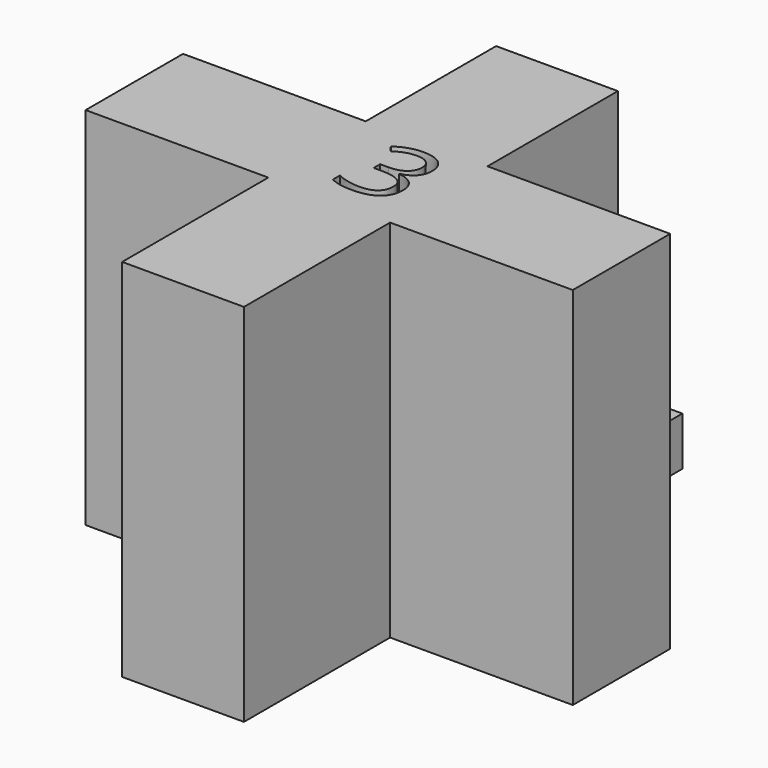
from build123d import *

# Parameters (mm, degrees)
F0_W         = 12.7
F0_H         = 57.15
F1_DEPTH     = 5.08
F2_W         = 50.8
F2_H         = 12.7
F3_DEPTH     = 38.1
F4_W         = 12.7
F4_H         = 48.7413735385
F5_DEPTH     = 33.02
F6_TEXT_SIZE = 12.0747026004
F7_DEPTH     = 2.54


# Not quite as in the source:
# - Text() gives the source's letters only with a copy of the font that has no kerning and outlines rounded to 1/6400 em; it was checked with that copy


with BuildPart() as f1:
    # F0 (on Top) → F1 (new body)
    with BuildSketch(Plane.XY):
        with Locations((-37.0165128261, 2.9978602284)):
            Rectangle(F0_W, F0_H)
    extrude(amount=F1_DEPTH)

    # F2 (on Top) → F3 (join)
    with BuildSketch(Plane.XY):
        with Locations((-37.0165128261, -0.1771397716)):
            Rectangle(F2_W, F2_H)
    extrude(amount=F3_DEPTH)

    # F4 (on face) → F5 (join)
    with BuildSketch(Plane.XY.offset(5.08)):
        with Locations((-37.0165128261, -1.2064530024)):
            Rectangle(F4_W, F4_H)
    extrude(amount=F5_DEPTH)

    # F6 (on face) → F7 (cut)
    with BuildSketch(Plane.XY.offset(38.1)):
        with Locations((-39.5974777639, -3.8714513648)):
            Text('3', F6_TEXT_SIZE, font='Open Sans', text_align=(TextAlign.LEFT, TextAlign.BOTTOM))
    extrude(amount=-F7_DEPTH, mode=Mode.SUBTRACT)


solid = f1.part
